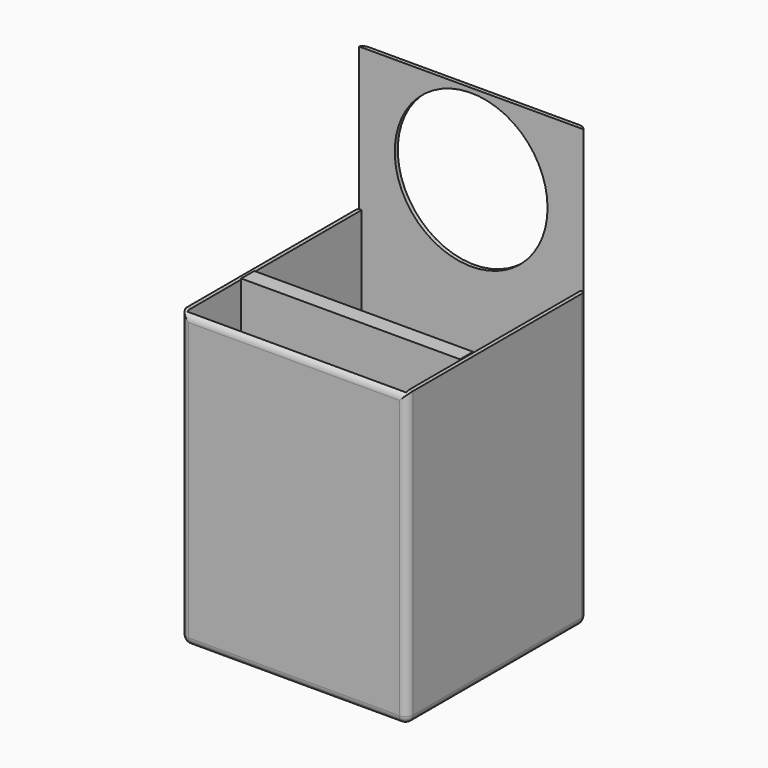
from build123d import *

# Parameters (mm, degrees)
F0_W         = 150.5279913545
F0_H         = 149.8499512672
F1_DEPTH     = 194.6834623814
F2_T         = -2.54
F3_W         = 2.54
F3_H         = 2.54
F4_DEPTH     = 95.1251834631
F6_D         = 101.6
F6_DEPTH     = 2.541
F7_T1_DEPTH  = 202.3034623814
F7_T3_DEPTH  = 297.4286458445
F7_T5_DEPTH  = 140.3679913545
F7_T7_DEPTH  = 139.6899512672
F7_T9_DEPTH  = 175.9279913545
F7_S13_W     = 5.08
F7_S13_H     = 5.08
F7_T14_DEPTH = 5.08
F7_S19_W     = 5.08
F7_S19_H     = 5.08
F7_T20_DEPTH = 5.08
F7_S25_W     = 5.08
F7_S25_H     = 5.08
F7_T26_DEPTH = 5.08
F7_S31_W     = 5.08
F7_S31_H     = 5.08
F7_T32_DEPTH = 5.08
F8_W         = 145.4479913545
F8_H         = 10.8655169606
F9_DEPTH     = 192.7349418402
F11_D        = 25.4
F11_DEPTH    = 12.7
F11_TIP      = 7.6309298617


# Not quite as in the source:
# - a fillet or chamfer that OpenCascade refuses, or shapes differently, is made with other operations: its cross-section is extruded or revolved along the edge and cut away or added


with BuildPart() as f1:
    # F0 (on Top) → F1 (new body)
    with BuildSketch(Plane.XY):
        with Locations((-0.0158064067, 0.4480481148)):
            Rectangle(F0_W, F0_H)
    extrude(amount=F1_DEPTH)

    # F2
    f2_openings = [f1.faces().sort_by_distance(p)[0] for p in [
        (-0.015806, 0.448048, 194.683462),
    ]]
    offset(amount=F2_T, openings=f2_openings)

    # F3 (on face) → F4 (join)
    with BuildSketch(Plane.XY.offset(194.6834623814)):
        Polygon((72.7081892705, 75.3730237484), (-75.279802084, 75.3730237484), (-75.279802084, 72.8330237484), (-72.739802084, 72.8330237484), (72.7081892705, 72.8330237484), align=None)
        with Locations((73.9781892705, 74.1030237484)):
            Rectangle(F3_W, F3_H)
    extrude(amount=F4_DEPTH)

    # F6 (through all, one way)
    with BuildSketch(Plane.XZ.offset(-72.8330237484)):
        with Locations((0, 236.040353775)):
            Circle(F6_D / 2)
    extrude(amount=-F6_DEPTH, mode=Mode.SUBTRACT)

    # F7: fillet of radius 5.08 on 9 edges, made by hand

    # F7_s2 → F7_t1 (cut)
    with BuildSketch(Plane.XY.offset(5.08)):
        with BuildLine():
            ThreePointArc((-75.279802084, -69.3969275188), (-73.7919045324, -72.9890299673), (-70.199802084, -74.4769275188))
            Line((-70.199802084, -74.4769275188), (-75.279802084, -74.4769275188))
            Line((-75.279802084, -74.4769275188), (-75.279802084, -69.3969275188))
        make_face()
        with BuildLine():
            ThreePointArc((75.2481892705, -69.3969275188), (73.7602917189, -72.9890299673), (70.1681892705, -74.4769275188))
            Line((70.1681892705, -74.4769275188), (75.2481892705, -74.4769275188))
            Line((75.2481892705, -74.4769275188), (75.2481892705, -69.3969275188))
        make_face()
    extrude(amount=F7_T1_DEPTH, mode=Mode.SUBTRACT)

    # F7_s4 → F7_t3 (cut)
    with BuildSketch(Plane.XY.offset(5.08)):
        with BuildLine():
            ThreePointArc((-70.199802084, 75.3730237484), (-73.7919045324, 73.8851261968), (-75.279802084, 70.2930237484))
            Line((-75.279802084, 70.2930237484), (-75.279802084, 75.3730237484))
            Line((-75.279802084, 75.3730237484), (-70.199802084, 75.3730237484))
        make_face()
        with BuildLine():
            ThreePointArc((70.1681892705, 75.3730237484), (73.7602917189, 73.8851261968), (75.2481892705, 70.2930237484))
            Line((75.2481892705, 70.2930237484), (75.2481892705, 75.3730237484))
            Line((75.2481892705, 75.3730237484), (70.1681892705, 75.3730237484))
        make_face()
    extrude(amount=F7_T3_DEPTH, mode=Mode.SUBTRACT)

    # F7_s6 → F7_t5 (cut)
    with BuildSketch(Plane.YZ.offset(-70.199802084)):
        with BuildLine():
            ThreePointArc((75.3730237484, 5.08), (73.8851261968, 1.4878975516), (70.2930237484, 0))
            Line((70.2930237484, 0), (75.3730237484, 0))
            Line((75.3730237484, 0), (75.3730237484, 5.08))
        make_face()
        with BuildLine():
            ThreePointArc((-69.3969275188, 0), (-72.9890299673, 1.4878975516), (-74.4769275188, 5.08))
            Line((-74.4769275188, 5.08), (-74.4769275188, 0))
            Line((-74.4769275188, 0), (-69.3969275188, 0))
        make_face()
    extrude(amount=F7_T5_DEPTH, mode=Mode.SUBTRACT)

    # F7_s8 → F7_t7 (cut)
    with BuildSketch(Plane.XZ.offset(-70.2930237484)):
        with BuildLine():
            ThreePointArc((-70.199802084, 0), (-73.7919045324, 1.4878975516), (-75.279802084, 5.08))
            Line((-75.279802084, 5.08), (-75.279802084, 0))
            Line((-75.279802084, 0), (-70.199802084, 0))
        make_face()
        with BuildLine():
            ThreePointArc((75.2481892705, 5.08), (73.7602917189, 1.4878975516), (70.1681892705, 0))
            Line((70.1681892705, 0), (75.2481892705, 0))
            Line((75.2481892705, 0), (75.2481892705, 5.08))
        make_face()
    extrude(amount=F7_T7_DEPTH, mode=Mode.SUBTRACT)

    # F7_s10 → F7_t9 (cut)
    with BuildSketch(Plane.YZ.offset(-87.979802084)):
        with BuildLine():
            ThreePointArc((-74.4769275188, 189.6034623814), (-72.9890299673, 193.1955648298), (-69.3969275188, 194.6834623814))
            Line((-69.3969275188, 194.6834623814), (-74.4769275188, 194.6834623814))
            Line((-74.4769275188, 194.6834623814), (-74.4769275188, 189.6034623814))
        make_face()
    extrude(amount=F7_T9_DEPTH, mode=Mode.SUBTRACT)


with BuildPart() as f7_tool12:
    # F7_s13 → F7_t14 (new body)
    with BuildSketch(Plane.XY.offset(5.08)):
        with Locations((-72.739802084, -71.9369275188)):
            Rectangle(F7_S13_W, F7_S13_H)
    extrude(amount=-F7_T14_DEPTH)

    # F7_s15 → F7_t16 (revolve, cut)
    with BuildSketch(Plane(origin=(-70.199802084, -69.3969275188, 5.08), x_dir=(0.7071067812, 0.7071067812, 0), z_dir=(-0.7071067812, 0.7071067812, 0))):
        with BuildLine():
            ThreePointArc((0, -5.08), (5.08, 0), (0, 5.08))
            Line((0, 5.08), (0, -5.08))
        make_face()
    revolve(axis=Axis((-70.199802084, -69.3969275188, 5.08), (0, 0, -1)), mode=Mode.SUBTRACT)


with BuildPart() as f1_1:
    add(f1.part)

    # F7_t11: cut F7_tool12
    add(f7_tool12.part, mode=Mode.SUBTRACT)


with BuildPart() as f7_tool18:
    # F7_s19 → F7_t20 (new body)
    with BuildSketch(Plane.XZ.offset(-70.2930237484)):
        with Locations((-72.739802084, 2.54)):
            Rectangle(F7_S19_W, F7_S19_H)
    extrude(amount=-F7_T20_DEPTH)

    # F7_s21 → F7_t22 (revolve, cut)
    with BuildSketch(Plane(origin=(-70.199802084, 70.2930237484, 5.08), x_dir=(0.7071067812, 0, 0.7071067812), z_dir=(-0.7071067812, 0, 0.7071067812))):
        with BuildLine():
            ThreePointArc((0, -5.08), (5.08, 0), (0, 5.08))
            Line((0, 5.08), (0, -5.08))
        make_face()
    revolve(axis=Axis((-70.199802084, 70.2930237484, 5.08), (0, 1, 0)), mode=Mode.SUBTRACT)


with BuildPart() as f1_2:
    add(f1_1.part)

    # F7_t17: cut F7_tool18
    add(f7_tool18.part, mode=Mode.SUBTRACT)


with BuildPart() as f7_tool24:
    # F7_s25 → F7_t26 (new body)
    with BuildSketch(Plane.XZ.offset(-70.2930237484)):
        with Locations((72.7081892705, 2.54)):
            Rectangle(F7_S25_W, F7_S25_H)
    extrude(amount=-F7_T26_DEPTH)

    # F7_s27 → F7_t28 (revolve, cut)
    with BuildSketch(Plane(origin=(70.1681892705, 70.2930237484, 5.08), x_dir=(-0.7071067812, 0, 0.7071067812), z_dir=(-0.7071067812, 0, -0.7071067812))):
        with BuildLine():
            ThreePointArc((0, -5.08), (5.08, 0), (0, 5.08))
            Line((0, 5.08), (0, -5.08))
        make_face()
    revolve(axis=Axis((70.1681892705, 70.2930237484, 5.08), (0, 1, 0)), mode=Mode.SUBTRACT)


with BuildPart() as f1_3:
    add(f1_2.part)

    # F7_t23: cut F7_tool24
    add(f7_tool24.part, mode=Mode.SUBTRACT)


with BuildPart() as f7_tool30:
    # F7_s31 → F7_t32 (new body)
    with BuildSketch(Plane.YZ.offset(70.1681892705)):
        with Locations((-71.9369275188, 2.54)):
            Rectangle(F7_S31_W, F7_S31_H)
    extrude(amount=F7_T32_DEPTH)

    # F7_s33 → F7_t34 (revolve, cut)
    with BuildSketch(Plane(origin=(70.1681892705, -69.3969275188, 5.08), x_dir=(0, 0.7071067812, 0.7071067812), z_dir=(0, 0.7071067812, -0.7071067812))):
        with BuildLine():
            ThreePointArc((0, -5.08), (5.08, 0), (0, 5.08))
            Line((0, 5.08), (0, -5.08))
        make_face()
    revolve(axis=Axis((70.1681892705, -69.3969275188, 5.08), (1, 0, 0)), mode=Mode.SUBTRACT)


with BuildPart() as f1_4:
    add(f1_3.part)

    # F7_t29: cut F7_tool30
    add(f7_tool30.part, mode=Mode.SUBTRACT)

    # F8 (on face) → F9 (join)
    with BuildSketch(Plane.XY.offset(2.54)):
        with Locations((-0.0158064067, -21.8428857625)):
            Rectangle(F8_W, F8_H)
    extrude(amount=F9_DEPTH)

    # F11 (one way)
    with BuildSketch(Plane.XZ.offset(27.2756442428)):
        with Locations((-4.689078778, 137.1918618679)):
            Circle(F11_D / 2)
    extrude(amount=-F11_DEPTH, mode=Mode.SUBTRACT)
    with Locations(Plane.XZ.offset(27.2756442428)):
        with Locations((-4.689078778, 137.1918618679)):
            with Locations((0, 0, -(F11_DEPTH + F11_TIP / 2))):  # 118° drill point
                Cone(0, F11_D / 2, F11_TIP, mode=Mode.SUBTRACT)


solid = f1_4.part
